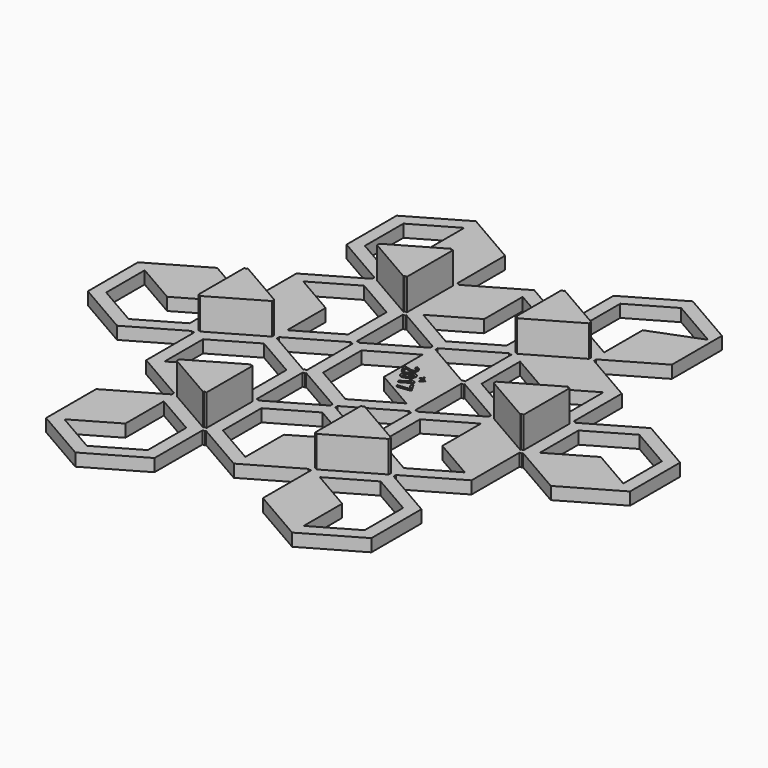
from build123d import *

# Parameters (mm, degrees)
F1_DEPTH       = 2.5
F2_DEPTH       = 15
F2_DEPTH_BACK  = 2
F3_TEXT_SIZE   = 7.1886174181
F3_TEXT_SIZE_2 = 3.2792485056
F4_DEPTH       = 1


# Not quite as in the source:
# - a feature names something its author has since deleted; it is built from what else it names
# - Text() gives the source's letters only with a copy of the font that has no kerning and outlines rounded to 1/6400 em; it was checked with that copy


with BuildPart() as f1:
    # F0 (on Top) → F1 (new body, symmetric)
    with BuildSketch(Plane.XY):
        Polygon((-22.6506350946, 13.5), (-21.6506350946, 13.5), (-21.6506350946, 36.5), (-22.6506350946, 36.5), (-22.6506350946, 38.0773502692), (-42.3012701892, 49.4226497308), (-42.3012701892, 49), (-44.3012701892, 49), (-44.3012701892, 49.4226497308), (-64.9519052838, 37.5), (-64.9519052838, 13.5), (-63.9519052838, 13.5), (-63.9519052838, 11.9226497308), (-44.3012701892, 0.5773502692), (-44.3012701892, 1), (-42.3012701892, 1), (-42.3012701892, 0.5773502692), (-22.6506350946, 11.9226497308), align=None)
        Polygon((-26.6506350946, 34.6132486541), (-26.6506350946, 15.3867513459), (-43.3012701892, 5.7735026919), (-43.3012701892, 25), (-59.9519052838, 34.6132486541), (-43.3012701892, 44.2264973081), align=None, mode=Mode.SUBTRACT)
        Polygon((-42.3012701892, 49), (-42.3012701892, 49.4226497308), (-43.3012701892, 50), (-44.3012701892, 49.4226497308), (-44.3012701892, 49), align=None)
        Polygon((-44.3012701892, 49.4226497308), (-43.3012701892, 50), (-44.3012701892, 50.5773502692), align=None)
        Polygon((-44.3012701892, 50.5773502692), (-43.3012701892, 50), (-42.3012701892, 50.5773502692), (-42.3012701892, 51), (-44.3012701892, 51), align=None)
        Polygon((-43.3012701892, 50), (-42.3012701892, 49.4226497308), (-42.3012701892, 50.5773502692), align=None)
        Polygon((-42.3012701892, 51), (-42.3012701892, 50.5773502692), (-22.6506350946, 61.9226497308), (-22.6506350946, 63.5), (-21.6506350946, 63.5), (-21.6506350946, 87.5), (-43.3012701892, 100), (-64.9519052838, 87.5), (-64.9519052838, 62.5), (-44.3012701892, 50.5773502692), (-44.3012701892, 51), align=None)
        Polygon((-59.9519052838, 65.3867513459), (-59.9519052838, 84.6132486541), (-43.3012701892, 94.2264973081), (-43.3012701892, 75), (-26.6506350946, 65.3867513459), (-43.3012701892, 55.7735026919), align=None, mode=Mode.SUBTRACT)
        Polygon((-21.6506350946, 37.5), (-20.6506350946, 36.9226497308), (-20.6506350946, 38.5), (-21.6506350946, 38.5), align=None)
        Polygon((1, 26), (1, 25.5773502692), (20.6506350946, 36.9226497308), (20.6506350946, 38.5), (21.6506350946, 38.5), (21.6506350946, 61.5), (20.6506350946, 61.5), (20.6506350946, 63.0773502692), (0, 75), (-20.6506350946, 63.0773502692), (-20.6506350946, 61.5), (-21.6506350946, 61.5), (-21.6506350946, 38.5), (-20.6506350946, 38.5), (-20.6506350946, 36.9226497308), (-1, 25.5773502692), (-1, 26), align=None)
        Polygon((16.6506350946, 40.3867513459), (0, 30.7735026919), (-16.6506350946, 40.3867513459), (0, 50), (0, 69.2264973081), (16.6506350946, 59.6132486541), align=None, mode=Mode.SUBTRACT)
        Polygon((-21.6506350946, 36.5), (-21.6506350946, 37.5), (-22.6506350946, 38.0773502692), (-22.6506350946, 36.5), align=None)
        Polygon((-20.6506350946, 36.5), (-20.6506350946, 36.9226497308), (-21.6506350946, 37.5), (-21.6506350946, 36.5), align=None)
        Polygon((-22.6506350946, 38.0773502692), (-21.6506350946, 37.5), (-21.6506350946, 38.5), (-22.6506350946, 38.5), align=None)
        Polygon((21.6506350946, -11.5), (21.6506350946, 11.5), (20.6506350946, 11.5), (20.6506350946, 13.0773502692), (1, 24.4226497308), (1, 24), (-1, 24), (-1, 24.4226497308), (-20.6506350946, 13.0773502692), (-20.6506350946, 11.5), (-21.6506350946, 11.5), (-21.6506350946, -11.5), (-20.6506350946, -11.5), (-20.6506350946, -13.0773502692), (-1, -24.4226497308), (-1, -24), (1, -24), (1, -24.4226497308), (20.6506350946, -13.0773502692), (20.6506350946, -11.5), align=None)
        Polygon((-16.6506350946, -9.6132486541), (-16.6506350946, 9.6132486541), (0, 19.2264973081), (0, 0), (16.6506350946, -9.6132486541), (0, -19.2264973081), align=None, mode=Mode.SUBTRACT)
        Polygon((-1, 25.5773502692), (0, 25), (1, 25.5773502692), (1, 26), (-1, 26), align=None)
        Polygon((1, 24), (1, 24.4226497308), (0, 25), (-1, 24.4226497308), (-1, 24), align=None)
        Polygon((-1, 24.4226497308), (0, 25), (-1, 25.5773502692), align=None)
        Polygon((0, 25), (1, 24.4226497308), (1, 25.5773502692), align=None)
        Polygon((-21.6506350946, 12.5), (-20.6506350946, 13.0773502692), (-20.6506350946, 13.5), (-21.6506350946, 13.5), align=None)
        Polygon((-22.6506350946, 11.9226497308), (-21.6506350946, 12.5), (-21.6506350946, 13.5), (-22.6506350946, 13.5), align=None)
        Polygon((-20.6506350946, 11.5), (-20.6506350946, 13.0773502692), (-21.6506350946, 12.5), (-21.6506350946, 11.5), align=None)
        Polygon((-21.6506350946, 11.5), (-21.6506350946, 12.5), (-22.6506350946, 11.9226497308), (-22.6506350946, 11.5), align=None)
        Polygon((21.6506350946, 13.5), (21.6506350946, 12.5), (22.6506350946, 11.9226497308), (22.6506350946, 13.5), align=None)
        Polygon((21.6506350946, 11.5), (21.6506350946, 12.5), (20.6506350946, 13.0773502692), (20.6506350946, 11.5), align=None)
        Polygon((22.6506350946, 11.9226497308), (21.6506350946, 12.5), (21.6506350946, 11.5), (22.6506350946, 11.5), align=None)
        Polygon((20.6506350946, 13.0773502692), (21.6506350946, 12.5), (21.6506350946, 13.5), (20.6506350946, 13.5), align=None)
        Polygon((21.6506350946, 37.5), (21.6506350946, 36.5), (22.6506350946, 36.5), (22.6506350946, 38.0773502692), align=None)
        Polygon((21.6506350946, 38.5), (21.6506350946, 37.5), (22.6506350946, 38.0773502692), (22.6506350946, 38.5), align=None)
        Polygon((20.6506350946, 36.9226497308), (21.6506350946, 37.5), (21.6506350946, 38.5), (20.6506350946, 38.5), align=None)
        Polygon((20.6506350946, 36.5), (21.6506350946, 36.5), (21.6506350946, 37.5), (20.6506350946, 36.9226497308), align=None)
        Polygon((43.3012701892, 50), (42.3012701892, 49.4226497308), (42.3012701892, 49), (44.3012701892, 49), (44.3012701892, 49.4226497308), align=None)
        Polygon((44.3012701892, 50.5773502692), (43.3012701892, 50), (44.3012701892, 49.4226497308), align=None)
        Polygon((42.3012701892, 50.5773502692), (43.3012701892, 50), (44.3012701892, 50.5773502692), (44.3012701892, 51), (42.3012701892, 51), align=None)
        Polygon((42.3012701892, 50.5773502692), (42.3012701892, 49.4226497308), (43.3012701892, 50), align=None)
        Polygon((22.6506350946, 61.9226497308), (42.3012701892, 50.5773502692), (42.3012701892, 51), (44.3012701892, 51), (44.3012701892, 50.5773502692), (64.9519052838, 62.5), (64.9519052838, 87.5), (43.3012701892, 100), (21.6506350946, 87.5), (21.6506350946, 63.5), (22.6506350946, 63.5), align=None)
        Polygon((26.6506350946, 84.6132486541), (43.3012701892, 94.2264973081), (63.2675009952, 82.6989885776), (43.3012701892, 75), (43.3012701892, 55.7735026919), (26.6506350946, 65.3867513459), align=None, mode=Mode.SUBTRACT)
        Polygon((21.6506350946, 63.5), (21.6506350946, 62.5), (22.6506350946, 61.9226497308), (22.6506350946, 63.5), align=None)
        Polygon((20.6506350946, 63.0773502692), (21.6506350946, 62.5), (21.6506350946, 63.5), (20.6506350946, 63.5), align=None)
        Polygon((20.6506350946, 61.5), (21.6506350946, 61.5), (21.6506350946, 62.5), (20.6506350946, 63.0773502692), align=None)
        Polygon((21.6506350946, 62.5), (21.6506350946, 61.5), (22.6506350946, 61.5), (22.6506350946, 61.9226497308), align=None)
        Polygon((65.9519052838, 11.5), (64.9519052838, 11.5), (64.9519052838, -11.5), (65.9519052838, -11.5), (65.9519052838, -13.0773502692), (86.6025403784, -25), (108.2531754731, -12.5), (108.2531754731, 12.5), (86.6025403784, 25), (65.9519052838, 13.0773502692), align=None)
        Polygon((86.6025403784, 19.2264973081), (103.2531754731, 9.6132486541), (103.2531754731, -9.6132486541), (86.6025403784, 0), (69.9519052838, -9.6132486541), (69.9519052838, 9.6132486541), align=None, mode=Mode.SUBTRACT)
        Polygon((65.9519052838, 13.0773502692), (64.9519052838, 12.5), (64.9519052838, 11.5), (65.9519052838, 11.5), align=None)
        Polygon((64.9519052838, 13.5), (64.9519052838, 12.5), (65.9519052838, 13.0773502692), (65.9519052838, 13.5), align=None)
        Polygon((63.9519052838, 13.5), (63.9519052838, 11.9226497308), (64.9519052838, 12.5), (64.9519052838, 13.5), align=None)
        Polygon((64.9519052838, 12.5), (63.9519052838, 11.9226497308), (63.9519052838, 11.5), (64.9519052838, 11.5), align=None)
        Polygon((44.3012701892, -0.5773502692), (43.3012701892, 0), (42.3012701892, -0.5773502692), (42.3012701892, -1), (44.3012701892, -1), align=None)
        Polygon((44.3012701892, 0.5773502692), (43.3012701892, 0), (44.3012701892, -0.5773502692), align=None)
        Polygon((42.3012701892, 1), (42.3012701892, 0.5773502692), (43.3012701892, 0), (44.3012701892, 0.5773502692), (44.3012701892, 1), align=None)
        Polygon((43.3012701892, 0), (42.3012701892, 0.5773502692), (42.3012701892, -0.5773502692), align=None)
        Polygon((64.9519052838, -12.5), (63.9519052838, -11.9226497308), (63.9519052838, -13.5), (64.9519052838, -13.5), align=None)
        Polygon((63.9519052838, -11.5), (63.9519052838, -11.9226497308), (64.9519052838, -12.5), (64.9519052838, -11.5), align=None)
        Polygon((64.9519052838, -11.5), (64.9519052838, -12.5), (65.9519052838, -13.0773502692), (65.9519052838, -11.5), align=None)
        Polygon((65.9519052838, -13.0773502692), (64.9519052838, -12.5), (64.9519052838, -13.5), (65.9519052838, -13.5), align=None)
        Polygon((21.6506350946, -13.5), (21.6506350946, -12.5), (20.6506350946, -13.0773502692), (20.6506350946, -13.5), align=None)
        Polygon((21.6506350946, -12.5), (21.6506350946, -11.5), (20.6506350946, -11.5), (20.6506350946, -13.0773502692), align=None)
        Polygon((22.6506350946, -11.9226497308), (21.6506350946, -12.5), (21.6506350946, -13.5), (22.6506350946, -13.5), align=None)
        Polygon((22.6506350946, -11.5), (21.6506350946, -11.5), (21.6506350946, -12.5), (22.6506350946, -11.9226497308), align=None)
        Polygon((22.6506350946, -36.5), (21.6506350946, -36.5), (21.6506350946, -37.5), (22.6506350946, -38.0773502692), align=None)
        Polygon((22.6506350946, -38.0773502692), (21.6506350946, -37.5), (21.6506350946, -38.5), (22.6506350946, -38.5), align=None)
        Polygon((21.6506350946, -37.5), (21.6506350946, -36.5), (20.6506350946, -36.5), (20.6506350946, -36.9226497308), align=None)
        Polygon((21.6506350946, -38.5), (21.6506350946, -37.5), (20.6506350946, -36.9226497308), (20.6506350946, -38.5), align=None)
        Polygon((20.6506350946, -36.9226497308), (1, -25.5773502692), (1, -26), (-1, -26), (-1, -25.5773502692), (-20.6506350946, -36.9226497308), (-20.6506350946, -38.5), (-21.6506350946, -38.5), (-21.6506350946, -61.5), (-20.6506350946, -61.5), (-20.6506350946, -63.0773502692), (0, -75), (20.6506350946, -63.0773502692), (20.6506350946, -61.5), (21.6506350946, -61.5), (21.6506350946, -38.5), (20.6506350946, -38.5), align=None)
        Polygon((-16.6506350946, -40.3867513459), (0, -30.7735026919), (16.531467789, -40.31795007), (0, -50), (0, -69.2264973081), (-16.6506350946, -59.6132486541), align=None, mode=Mode.SUBTRACT)
        Polygon((1, -25.5773502692), (0, -25), (-1, -25.5773502692), (-1, -26), (1, -26), align=None)
        Polygon((-1, -25.5773502692), (0, -25), (-1, -24.4226497308), align=None)
        Polygon((1, -25.5773502692), (1, -24.4226497308), (0, -25), align=None)
        Polygon((0, -25), (1, -24.4226497308), (1, -24), (-1, -24), (-1, -24.4226497308), align=None)
        Polygon((-21.6506350946, -12.5), (-20.6506350946, -13.0773502692), (-20.6506350946, -11.5), (-21.6506350946, -11.5), align=None)
        Polygon((-20.6506350946, -13.5), (-20.6506350946, -13.0773502692), (-21.6506350946, -12.5), (-21.6506350946, -13.5), align=None)
        Polygon((-21.6506350946, -13.5), (-21.6506350946, -12.5), (-22.6506350946, -11.9226497308), (-22.6506350946, -13.5), align=None)
        Polygon((-21.6506350946, -12.5), (-21.6506350946, -11.5), (-22.6506350946, -11.5), (-22.6506350946, -11.9226497308), align=None)
        Polygon((-22.6506350946, -11.9226497308), (-42.3012701892, -0.5773502692), (-42.3012701892, -1), (-44.3012701892, -1), (-44.3012701892, -0.5773502692), (-63.9519052838, -11.9226497308), (-63.9519052838, -13.5), (-64.9519052838, -13.5), (-64.9519052838, -37.5), (-44.3012701892, -49.4226497308), (-44.3012701892, -49), (-42.3012701892, -49), (-42.3012701892, -49.4226497308), (-22.6506350946, -38.0773502692), (-22.6506350946, -36.5), (-21.6506350946, -36.5), (-21.6506350946, -13.5), (-22.6506350946, -13.5), align=None)
        Polygon((-43.3012701892, -5.7735026919), (-26.6506350946, -15.3867513459), (-26.6506350946, -34.6132486541), (-43.3012701892, -25), (-59.9519052838, -34.6132486541), (-59.9519052838, -15.3867513459), align=None, mode=Mode.SUBTRACT)
        Polygon((-22.6506350946, -38.0773502692), (-21.6506350946, -37.5), (-21.6506350946, -36.5), (-22.6506350946, -36.5), align=None)
        Polygon((-21.6506350946, -37.5), (-20.6506350946, -36.9226497308), (-20.6506350946, -36.5), (-21.6506350946, -36.5), align=None)
        Polygon((-20.6506350946, -38.5), (-20.6506350946, -36.9226497308), (-21.6506350946, -37.5), (-21.6506350946, -38.5), align=None)
        Polygon((-21.6506350946, -38.5), (-21.6506350946, -37.5), (-22.6506350946, -38.0773502692), (-22.6506350946, -38.5), align=None)
        Polygon((42.3012701892, -51), (42.3012701892, -50.5773502692), (22.6506350946, -61.9226497308), (22.6506350946, -63.5), (21.6506350946, -63.5), (21.6506350946, -87.5), (43.3012701892, -100), (64.9519052838, -87.5), (64.9519052838, -62.5), (44.3012701892, -50.5773502692), (44.3012701892, -51), align=None)
        Polygon((59.9519052838, -65.3867513459), (59.9519052838, -84.6132486541), (43.3012701892, -94.2264973081), (43.3012701892, -75), (26.6506350946, -65.3867513459), (43.3012701892, -55.7735026919), align=None, mode=Mode.SUBTRACT)
        Polygon((44.3012701892, -50.5773502692), (43.3012701892, -50), (42.3012701892, -50.5773502692), (42.3012701892, -51), (44.3012701892, -51), align=None)
        Polygon((44.3012701892, -49.4226497308), (43.3012701892, -50), (44.3012701892, -50.5773502692), align=None)
        Polygon((42.3012701892, -49), (42.3012701892, -49.4226497308), (43.3012701892, -50), (44.3012701892, -49.4226497308), (44.3012701892, -49), align=None)
        Polygon((43.3012701892, -50), (42.3012701892, -49.4226497308), (42.3012701892, -50.5773502692), align=None)
        Polygon((22.6506350946, -61.9226497308), (21.6506350946, -62.5), (21.6506350946, -63.5), (22.6506350946, -63.5), align=None)
        Polygon((22.6506350946, -61.5), (21.6506350946, -61.5), (21.6506350946, -62.5), (22.6506350946, -61.9226497308), align=None)
        Polygon((21.6506350946, -62.5), (21.6506350946, -61.5), (20.6506350946, -61.5), (20.6506350946, -63.0773502692), align=None)
        Polygon((21.6506350946, -63.5), (21.6506350946, -62.5), (20.6506350946, -63.0773502692), (20.6506350946, -63.5), align=None)
        Polygon((-20.6506350946, -61.5), (-21.6506350946, -61.5), (-21.6506350946, -62.5), (-20.6506350946, -63.0773502692), align=None)
        Polygon((-20.6506350946, -63.0773502692), (-21.6506350946, -62.5), (-21.6506350946, -63.5), (-20.6506350946, -63.5), align=None)
        Polygon((-21.6506350946, -63.5), (-21.6506350946, -62.5), (-22.6506350946, -61.9226497308), (-22.6506350946, -63.5), align=None)
        Polygon((-21.6506350946, -62.5), (-21.6506350946, -61.5), (-22.6506350946, -61.5), (-22.6506350946, -61.9226497308), align=None)
        Polygon((-22.6506350946, -61.9226497308), (-42.3012701892, -50.5773502692), (-42.3012701892, -51), (-44.3012701892, -51), (-44.3012701892, -50.5773502692), (-64.9519052838, -62.5), (-64.9519052838, -87.5), (-43.3012701892, -100), (-21.6506350946, -87.5), (-21.6506350946, -63.5), (-22.6506350946, -63.5), align=None)
        Polygon((-26.6506350946, -84.6132486541), (-43.3012701892, -94.2264973081), (-59.9519052838, -84.6132486541), (-43.3012701892, -75), (-43.3012701892, -55.7735026919), (-26.6506350946, -65.3867513459), align=None, mode=Mode.SUBTRACT)
        Polygon((-42.3012701892, -50.5773502692), (-43.3012701892, -50), (-44.3012701892, -50.5773502692), (-44.3012701892, -51), (-42.3012701892, -51), align=None)
        Polygon((-42.3012701892, -50.5773502692), (-42.3012701892, -49.4226497308), (-43.3012701892, -50), align=None)
        Polygon((-43.3012701892, -50), (-42.3012701892, -49.4226497308), (-42.3012701892, -49), (-44.3012701892, -49), (-44.3012701892, -49.4226497308), align=None)
        Polygon((-44.3012701892, -50.5773502692), (-43.3012701892, -50), (-44.3012701892, -49.4226497308), align=None)
        Polygon((-63.9519052838, -13.5), (-63.9519052838, -11.9226497308), (-64.9519052838, -12.5), (-64.9519052838, -13.5), align=None)
        Polygon((-64.9519052838, -13.5), (-64.9519052838, -12.5), (-65.9519052838, -13.0773502692), (-65.9519052838, -13.5), align=None)
        Polygon((-65.9519052838, -13.0773502692), (-64.9519052838, -12.5), (-64.9519052838, -11.5), (-65.9519052838, -11.5), align=None)
        Polygon((-64.9519052838, -12.5), (-63.9519052838, -11.9226497308), (-63.9519052838, -11.5), (-64.9519052838, -11.5), align=None)
        Polygon((-65.9519052838, -11.5), (-64.9519052838, -11.5), (-64.9519052838, 11.5), (-65.9519052838, 11.5), (-65.9519052838, 13.0773502692), (-86.6025403784, 25), (-108.2531754731, 12.5), (-108.2531754731, -12.5), (-86.6025403784, -25), (-65.9519052838, -13.0773502692), align=None)
        Polygon((-86.6025403784, -19.2264973081), (-103.2531754731, -9.6132486541), (-103.2531754731, 9.613248654), (-86.6025403784, 0), (-69.9519052838, 9.6132486541), (-69.9519052838, -9.6132486541), align=None, mode=Mode.SUBTRACT)
        Polygon((-42.3012701892, -0.5773502692), (-43.3012701892, 0), (-44.3012701892, -0.5773502692), (-44.3012701892, -1), (-42.3012701892, -1), align=None)
        Polygon((-43.3012701892, 0), (-42.3012701892, 0.5773502692), (-42.3012701892, 1), (-44.3012701892, 1), (-44.3012701892, 0.5773502692), align=None)
        Polygon((-42.3012701892, -0.5773502692), (-42.3012701892, 0.5773502692), (-43.3012701892, 0), align=None)
        Polygon((-44.3012701892, -0.5773502692), (-43.3012701892, 0), (-44.3012701892, 0.5773502692), align=None)
        Polygon((-63.9519052838, 11.5), (-63.9519052838, 11.9226497308), (-64.9519052838, 12.5), (-64.9519052838, 11.5), align=None)
        Polygon((-64.9519052838, 12.5), (-63.9519052838, 11.9226497308), (-63.9519052838, 13.5), (-64.9519052838, 13.5), align=None)
        Polygon((-65.9519052838, 13.0773502692), (-64.9519052838, 12.5), (-64.9519052838, 13.5), (-65.9519052838, 13.5), align=None)
        Polygon((-64.9519052838, 11.5), (-64.9519052838, 12.5), (-65.9519052838, 13.0773502692), (-65.9519052838, 11.5), align=None)
        Polygon((-22.6506350946, 61.9226497308), (-21.6506350946, 62.5), (-21.6506350946, 63.5), (-22.6506350946, 63.5), align=None)
        Polygon((-21.6506350946, 63.5), (-21.6506350946, 62.5), (-20.6506350946, 63.0773502692), (-20.6506350946, 63.5), align=None)
        Polygon((-22.6506350946, 61.5), (-21.6506350946, 61.5), (-21.6506350946, 62.5), (-22.6506350946, 61.9226497308), align=None)
        Polygon((-21.6506350946, 62.5), (-21.6506350946, 61.5), (-20.6506350946, 61.5), (-20.6506350946, 63.0773502692), align=None)
        Polygon((22.6506350946, 13.5), (22.6506350946, 11.9226497308), (42.3012701892, 0.5773502692), (42.3012701892, 1), (44.3012701892, 1), (44.3012701892, 0.5773502692), (63.9519052838, 11.9226497308), (63.9519052838, 13.5), (64.9519052838, 13.5), (64.9519052838, 37.5), (44.3012701892, 49.4226497308), (44.3012701892, 49), (42.3012701892, 49), (42.3012701892, 49.4226497308), (22.6506350946, 38.0773502692), (22.6506350946, 36.5), (21.6506350946, 36.5), (21.6506350946, 13.5), align=None)
        Polygon((43.3012701892, 5.7735026919), (26.6506350946, 15.3867513459), (26.6506350946, 34.6132486541), (43.3012701892, 25), (59.9519052838, 34.6132486541), (59.9519052838, 15.3867513459), align=None, mode=Mode.SUBTRACT)
        Polygon((42.3012701892, -1), (42.3012701892, -0.5773502692), (22.6506350946, -11.9226497308), (22.6506350946, -13.5), (21.6506350946, -13.5), (21.6506350946, -36.5), (22.6506350946, -36.5), (22.6506350946, -38.0773502692), (42.3012701892, -49.4226497308), (42.3012701892, -49), (44.3012701892, -49), (44.3012701892, -49.4226497308), (64.9519052838, -37.5), (64.9519052838, -13.5), (63.9519052838, -13.5), (63.9519052838, -11.9226497308), (44.3012701892, -0.5773502692), (44.3012701892, -1), align=None)
        Polygon((26.6506350946, -34.6132486541), (26.6506350946, -15.3867513459), (43.3012701892, -5.7735026919), (43.3012701892, -25), (59.9519052838, -34.6132486541), (43.3012701892, -44.2264973081), align=None, mode=Mode.SUBTRACT)
    extrude(amount=F1_DEPTH, both=True)

    # F3 (on face) → F4 (cut)
    with BuildSketch(Plane.XY.offset(2.5)):
        with Locations(Location((0, 9.6132486541), (0, 0, -60))):
            Text('2017', F3_TEXT_SIZE, font='Open Sans', font_style=FontStyle.BOLD, text_align=(TextAlign.LEFT, TextAlign.BOTTOM))
        with Locations(Location((8.8020702824, 6.8329437636), (0, 0, -60))):
            Text('v1', F3_TEXT_SIZE_2, font='Open Sans', text_align=(TextAlign.LEFT, TextAlign.BOTTOM))
    extrude(amount=-F4_DEPTH, mode=Mode.SUBTRACT)


with BuildPart() as f2:
    # F0 (on Top) → F2 (new body, two sides)
    with BuildSketch(Plane.XY) as f2_sk:
        Polygon((-42.3012701892, 49.4226497308), (-22.6506350946, 38.0773502692), (-22.6506350946, 38.5), (-21.6506350946, 38.5), (-21.6506350946, 61.5), (-22.6506350946, 61.5), (-22.6506350946, 61.9226497308), (-42.3012701892, 50.5773502692), align=None)
    extrude(amount=F2_DEPTH)
    extrude(f2_sk.sketch, amount=-F2_DEPTH_BACK)


with BuildPart() as f2b:
    # F0 (on Top) → F2, piece 2 (new body, two sides)
    with BuildSketch(Plane.XY) as f2_2_sk:
        Polygon((21.6506350946, 61.5), (21.6506350946, 38.5), (22.6506350946, 38.5), (22.6506350946, 38.0773502692), (42.3012701892, 49.4226497308), (42.3012701892, 50.5773502692), (22.6506350946, 61.9226497308), (22.6506350946, 61.5), align=None)
    extrude(amount=F2_DEPTH)
    extrude(f2_2_sk.sketch, amount=-F2_DEPTH_BACK)


with BuildPart() as f2c:
    # F0 (on Top) → F2, piece 3 (new body, two sides)
    with BuildSketch(Plane.XY) as f2_3_sk:
        Polygon((63.9519052838, 11.9226497308), (44.3012701892, 0.5773502692), (44.3012701892, -0.5773502692), (63.9519052838, -11.9226497308), (63.9519052838, -11.5), (64.9519052838, -11.5), (64.9519052838, 11.5), (63.9519052838, 11.5), align=None)
    extrude(amount=F2_DEPTH)
    extrude(f2_3_sk.sketch, amount=-F2_DEPTH_BACK)


with BuildPart() as f2d:
    # F0 (on Top) → F2, piece 4 (new body, two sides)
    with BuildSketch(Plane.XY) as f2_4_sk:
        Polygon((22.6506350946, -38.5), (21.6506350946, -38.5), (21.6506350946, -61.5), (22.6506350946, -61.5), (22.6506350946, -61.9226497308), (42.3012701892, -50.5773502692), (42.3012701892, -49.4226497308), (22.6506350946, -38.0773502692), align=None)
    extrude(amount=F2_DEPTH)
    extrude(f2_4_sk.sketch, amount=-F2_DEPTH_BACK)


with BuildPart() as f2e:
    # F0 (on Top) → F2, piece 5 (new body, two sides)
    with BuildSketch(Plane.XY) as f2_5_sk:
        Polygon((-21.6506350946, -61.5), (-21.6506350946, -38.5), (-22.6506350946, -38.5), (-22.6506350946, -38.0773502692), (-42.3012701892, -49.4226497308), (-42.3012701892, -50.5773502692), (-22.6506350946, -61.9226497308), (-22.6506350946, -61.5), align=None)
    extrude(amount=F2_DEPTH)
    extrude(f2_5_sk.sketch, amount=-F2_DEPTH_BACK)


with BuildPart() as f2f:
    # F0 (on Top) → F2, piece 6 (new body, two sides)
    with BuildSketch(Plane.XY) as f2_6_sk:
        Polygon((-63.9519052838, -11.9226497308), (-44.3012701892, -0.5773502692), (-44.3012701892, 0.5773502692), (-63.9519052838, 11.9226497308), (-63.9519052838, 11.5), (-64.9519052838, 11.5), (-64.9519052838, -11.5), (-63.9519052838, -11.5), align=None)
    extrude(amount=F2_DEPTH)
    extrude(f2_6_sk.sketch, amount=-F2_DEPTH_BACK)


solid = Compound([f1.part, f2.part, f2b.part, f2c.part, f2d.part, f2e.part, f2f.part])
